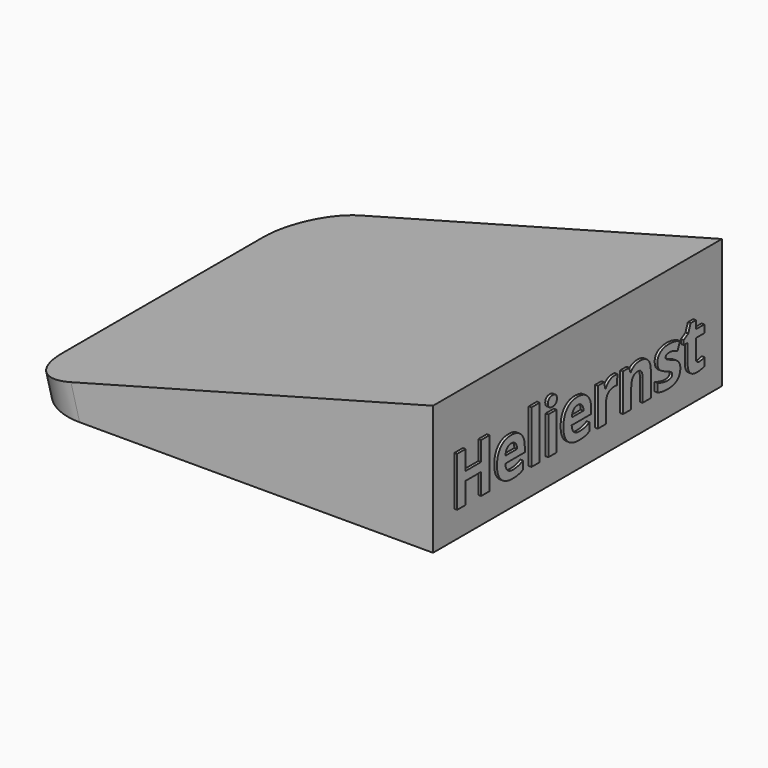
from build123d import *

# Parameters (mm, degrees)
F1_DEPTH     = 39.5
F4_ANGLE     = 90
F5_ANGLE     = 180
F6_TEXT_SIZE = 7.5560802834
F7_DEPTH     = 0.3
F1_FACE2_W   = 39.5
F1_FACE2_H   = 2
F9_DEPTH     = 13.7604974886


# Not quite as in the source:
# - Text() gives the source's letters only with a copy of the font that has no kerning and outlines rounded to 1/6400 em; it was checked with that copy


with BuildPart() as f1:
    # F0 (on Right) → F1 (new body)
    with BuildSketch(Plane.YZ):
        Polygon((0, 2), (0, 0), (45.3985138356, 0), (45.3985138356, 14.1644951198), align=None)
    extrude(amount=F1_DEPTH)


with BuildPart() as f2_1:
    # F2: copy of F1
    add(f1.part.moved(Location((-10.75, -78, 41.5))))


with BuildPart() as f1_1:
    # F4: moved
    add(f1.part.rotate(Axis((0, 45.3985138356, 7.0822475599), (0, 0, 1)), F4_ANGLE))


with BuildPart() as f1_2:
    # F5: moved
    add(f1_1.part.rotate(Axis((0, 45.3985138356, 7.0822475599), (0, 0, 1)), F5_ANGLE))

    # F6 (on face) → F7 (join)
    with BuildSketch(Plane.YZ):
        with Locations((8.1485138356, 3.0427512372)):
            Text('Heliernst', F6_TEXT_SIZE, font='Open Sans', font_style=FontStyle.BOLD, text_align=(TextAlign.LEFT, TextAlign.BOTTOM))
    extrude(amount=F7_DEPTH)

    # F8 (on face) + F1_face2 (on face) → F9 (cut, through all)
    with BuildSketch(Plane(origin=(-3.54112378, 0, 13.2156538627), x_dir=(0.9659258263, 0, 0.2588190451), z_dir=(-0.2588190451, 0, 0.9659258263))):
        with BuildLine():
            ThreePointArc((-43.3339588987, 39.3985138356), (-41.5765995858, 43.6411545227), (-37.3339588987, 45.3985138356))
            Line((-37.3339588987, 45.3985138356), (-43.3339588987, 45.3985138356))
            Line((-43.3339588987, 45.3985138356), (-43.3339588987, 39.3985138356))
        make_face()
        with BuildLine():
            ThreePointArc((-37.3339588987, 5.8985138356), (-41.5765995858, 7.6558731485), (-43.3339588987, 11.8985138356))
            Line((-43.3339588987, 11.8985138356), (-43.3339588987, 5.8985138356))
            Line((-43.3339588987, 5.8985138356), (-37.3339588987, 5.8985138356))
        make_face()
    with BuildSketch(Plane(origin=(-45.3985138356, 25.6485138356, 1), x_dir=(0, -1, 0), z_dir=(-1, 0, 0))):
        Rectangle(F1_FACE2_W, F1_FACE2_H)
    extrude(amount=-F9_DEPTH, dir=(-0.2588190451, 0, 0.9659258263), mode=Mode.SUBTRACT)


solid = f1_2.part
